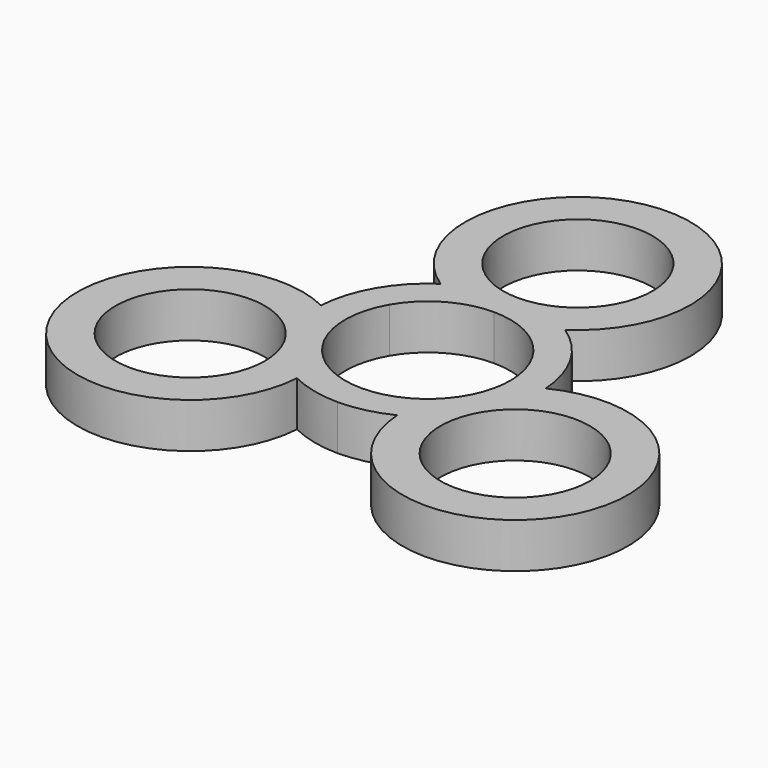
from build123d import *

# Parameters (mm, degrees)
F0_R     = 9.95
F1_DEPTH = 6


# Not quite as in the source:
# - a feature names something its author has since deleted; it is built from what else it names


with BuildPart() as f1:
    # F0 (on Top) → F1 (new body)
    with BuildSketch(Plane.XY):
        with BuildLine():
            ThreePointArc((8.2915619759, 12.5), (0, 40), (-8.2915619759, 12.5))
            ThreePointArc((-8.2915619759, 12.5), (-10.9307033082, 10.2722794544), (-12.9903810568, 7.5))
            ThreePointArc((-12.9903810568, 7.5), (-14.3614066163, 4.3301270189), (-14.9710985352, 0.9307033082))
            ThreePointArc((-14.9710985352, 0.9307033082), (-34.6410161514, -20), (-6.6795365594, -13.4307033082))
            ThreePointArc((-6.6795365594, -13.4307033082), (-3.4307033082, -14.6024064733), (0, -15))
            ThreePointArc((0, -15), (3.4307033082, -14.6024064733), (6.6795365594, -13.4307033082))
            ThreePointArc((6.6795365594, -13.4307033082), (34.6410161514, -20), (14.9710985352, 0.9307033082))
            ThreePointArc((14.9710985352, 0.9307033082), (14.3614066163, 4.3301270189), (12.9903810568, 7.5))
            ThreePointArc((12.9903810568, 7.5), (10.9307033082, 10.2722794544), (8.2915619759, 12.5))
        make_face()
        with Locations((-21.6506350946, -12.5)):
            Circle(F0_R, mode=Mode.SUBTRACT)
        with Locations((21.6506350946, -12.5)):
            Circle(F0_R, mode=Mode.SUBTRACT)
        with BuildLine():
            ThreePointArc((0, 11), (5.5, 9.5262794416), (9.5262794416, 5.5))
            ThreePointArc((9.5262794416, 5.5), (9.5262794416, -5.5), (0, -11))
            ThreePointArc((0, -11), (-9.5262794416, -5.5), (-9.5262794416, 5.5))
            ThreePointArc((-9.5262794416, 5.5), (-5.5, 9.5262794416), (0, 11))
        make_face(mode=Mode.SUBTRACT)
        with BuildLine():
            ThreePointArc((9.95, 25), (7.0357124728, 17.9642875272), (0, 15.05))
            ThreePointArc((0, 15.05), (-7.0357124728, 32.0357124728), (9.95, 25))
        make_face(mode=Mode.SUBTRACT)
    extrude(amount=F1_DEPTH)


solid = f1.part
